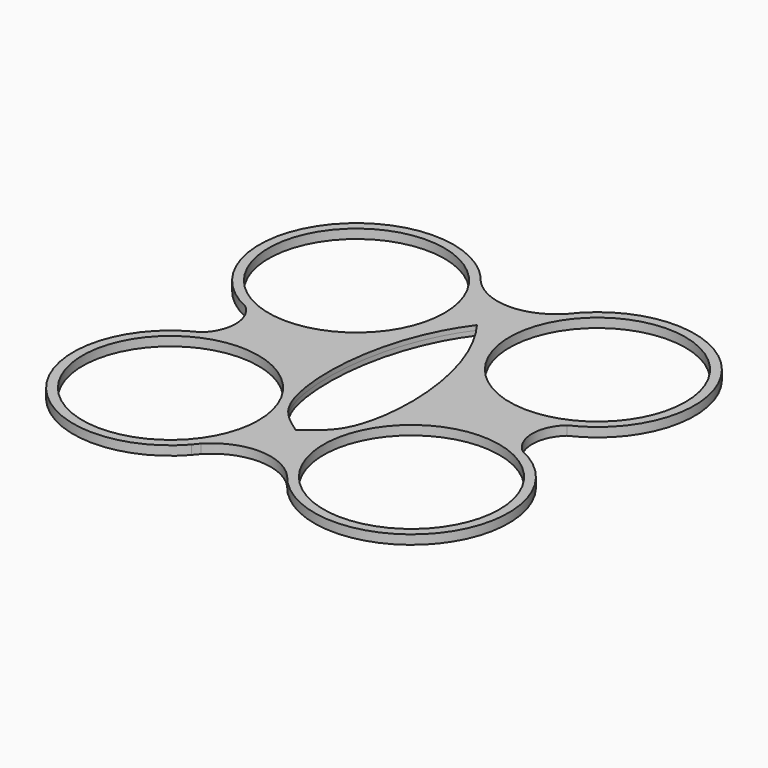
from build123d import *

# Parameters (mm, degrees)
F0_R     = 60.541459453
F2_DEPTH = 3.175


# Not quite as in the source:
# - the program builds the solid bodies; features that only make, move or delete a surface that nothing else refers to are left out


with BuildPart() as f2:
    # F0 (on Top) → F2 (new body, symmetric)
    with BuildSketch(Plane.XY):
        with BuildLine():
            ThreePointArc((29.63795994, 120.4253280383), (0, 107.6024649325), (-29.63795994, 120.4253280383))
            ThreePointArc((-29.63795994, 120.4253280383), (-31.4004725935, 122.4295872496), (-33.0277066154, 124.5451522517))
            ThreePointArc((-33.0277066154, 124.5451522517), (-136.833025163, 119.6500101861), (-110.5775391502, 19.1007385387))
            ThreePointArc((-110.5775391502, 19.1007385387), (-102.1103333636, 0), (-110.5775391502, -19.1007385387))
            ThreePointArc((-110.5775391502, -19.1007385387), (-136.833025163, -119.6500101861), (-33.0277066154, -124.5451522517))
            ThreePointArc((-33.0277066154, -124.5451522517), (-31.4004725935, -122.4295872496), (-29.63795994, -120.4253280383))
            ThreePointArc((-29.63795994, -120.4253280383), (0, -107.6024649325), (29.63795994, -120.4253280383))
            ThreePointArc((29.63795994, -120.4253280383), (135.2096998467, -121.7674331009), (110.5775391502, -19.1007385387))
            ThreePointArc((110.5775391502, -19.1007385387), (102.1103333636, 0), (110.5775391502, 19.1007385387))
            ThreePointArc((110.5775391502, 19.1007385387), (135.2096998467, 121.7674331009), (29.63795994, 120.4253280383))
        make_face()
        with Locations((-82.9460425302, -80.0184514167)):
            Circle(F0_R, mode=Mode.SUBTRACT)
        with Locations((82.9460425302, -80.0184514167)):
            Circle(F0_R, mode=Mode.SUBTRACT)
        with BuildLine():
            add(Edge.make_bspline(
                [(0, -76.0996581864), (9.5787021029, -69.2053000853), (33.1312215182, -54.3582389446), (31.8321399477, 37.4809793102), (0, 80.0184514167)],
                knots=[0, 0, 0, 0, 0.3369505381, 1, 1, 1, 1], degree=3))
            add(Edge.make_bspline(
                [(0, -76.0996581864), (-9.5787021029, -69.2053000853), (-33.1312215182, -54.3582389446), (-31.8321399477, 37.4809793102), (0, 80.0184514167)],
                knots=[0, 0, 0, 0, 0.3369505381, 1, 1, 1, 1], degree=3))
        make_face(mode=Mode.SUBTRACT)
        with Locations((-82.9460425302, 80.0184514167)):
            Circle(F0_R, mode=Mode.SUBTRACT)
        with Locations((82.9460425302, 80.0184514167)):
            Circle(F0_R, mode=Mode.SUBTRACT)
    extrude(amount=F2_DEPTH, both=True)


solid = f2.part
